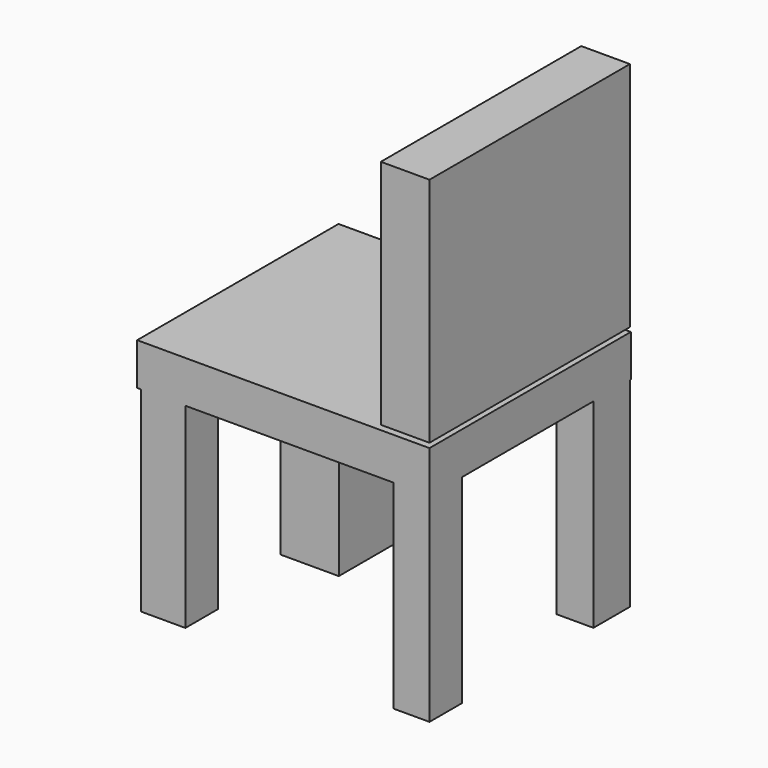
from build123d import *

# Parameters (mm, degrees)
F0_W      = 56.4791858196
F0_H      = 48.6274659634
F1_DEPTH  = 8.128
F2_W      = 8.5997208953
F2_H      = 37.7997383475
F2_W_2    = 6.992766168
F2_H_2    = 38.4415946901
F3_DEPTH  = 7.874
F4_W      = 8.7898299098
F4_H      = 38.5400280356
F5_DEPTH  = 7.112
F6_W      = 11.2653039396
F6_H      = 14.0175670385
F7_DEPTH  = 42.418
F8_W      = 48.401452601
F8_H      = 44.7438852862
F10_DEPTH = 9.398


# Not quite as in the source:
# - a feature of the source that left no trace in its solid (it failed there, or was rolled back) is left out


with BuildPart() as f1:
    # F0 (on Top) → F1 (new body)
    with BuildSketch(Plane.XY):
        with Locations((-28.2395929098, 24.3137329817)):
            Rectangle(F0_W, F0_H)
    extrude(amount=F1_DEPTH)

    # F2 (on Front) → F3 (join)
    with BuildSketch(Plane.XZ):
        with Locations((-51.4646843076, -18.8998691738)):
            Rectangle(F2_W, F2_H)
        with Locations((-3.496383084, -19.220797345)):
            Rectangle(F2_W_2, F2_H_2)
    extrude(amount=-F3_DEPTH)

    # F4 (on Right) → F5 (join)
    with BuildSketch(Plane.YZ):
        with Locations((43.9947880805, -19.2700140178)):
            Rectangle(F4_W, F4_H)
    extrude(amount=-F5_DEPTH)

    # F6 (on face) → F7 (join)
    with BuildSketch(Plane(origin=(0, 0, 0), x_dir=(1, 0, 0), z_dir=(0, 0, -1))):
        with Locations((-50.8465338498, -41.6186824441)):
            Rectangle(F6_W, F6_H)
    extrude(amount=F7_DEPTH)


with BuildPart() as f10:
    # F8 (on Right) → F10 (new body)
    with BuildSketch(Plane.YZ):
        with Locations((24.2007263005, 31.4088850282)):
            Rectangle(F8_W, F8_H)
    extrude(amount=-F10_DEPTH)


solid = Compound([f1.part, f10.part])
